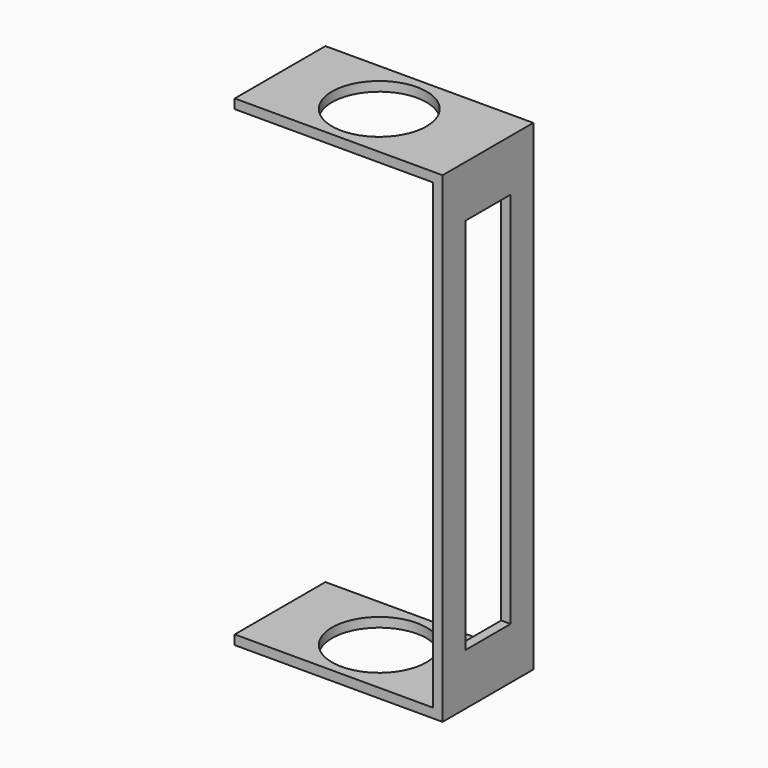
from build123d import *

# Parameters (mm, degrees)
F1_DEPTH       = 15.24
F4_D           = 12.7
F4_DEPTH       = 1.271
F4_ON_F2_D     = 12.7
F4_ON_F2_DEPTH = 1.271
F5_W           = 7.62
F5_H           = 25.4
F6_DEPTH       = 25.4


# Not quite as in the source:
# - a feature names something its author has since deleted; it is built from what else it names


with BuildPart() as f1:
    # F0 (on Front) → F1 (new body)
    with BuildSketch(Plane.XZ):
        Polygon((-14.4720045709, -37.1843738795), (13.4679954291, -37.1843738795), (13.4679954291, 27.5043461205), (-14.4720045709, 27.5043461205), (-14.4720045709, 26.2343461205), (12.1979954291, 26.2343461205), (12.1979954291, -35.9143738795), (-14.4720045709, -35.9143738795), align=None)
    extrude(amount=F1_DEPTH)

    # F4 (through all, one way)
    with BuildSketch(Plane.XY.offset(-35.9143738795)):
        with Locations((-1.1370045709, -7.62)):
            Circle(F4_D / 2)
    extrude(amount=-F4_DEPTH, mode=Mode.SUBTRACT)

    # F4 on F2 (through all, one way)
    with BuildSketch(Plane(origin=(0, 0, 26.2343461205), x_dir=(1, 0, 0), z_dir=(0, 0, -1))):
        with Locations((-1.1370045709, 7.62)):
            Circle(F4_ON_F2_D / 2)
    extrude(amount=-F4_ON_F2_DEPTH, mode=Mode.SUBTRACT)

    # F5 (on face) → F6 (cut)
    with BuildSketch(Plane(origin=(12.1979954291, 0, 0), x_dir=(0, -1, 0), z_dir=(-1, 0, 0))):
        with Locations((7.62, -17.5400138795)):
            Rectangle(F5_W, F5_H)
        with Locations((7.62, 7.8599861205)):
            Rectangle(F5_W, F5_H)
    extrude(amount=-F6_DEPTH, mode=Mode.SUBTRACT)


solid = f1.part
